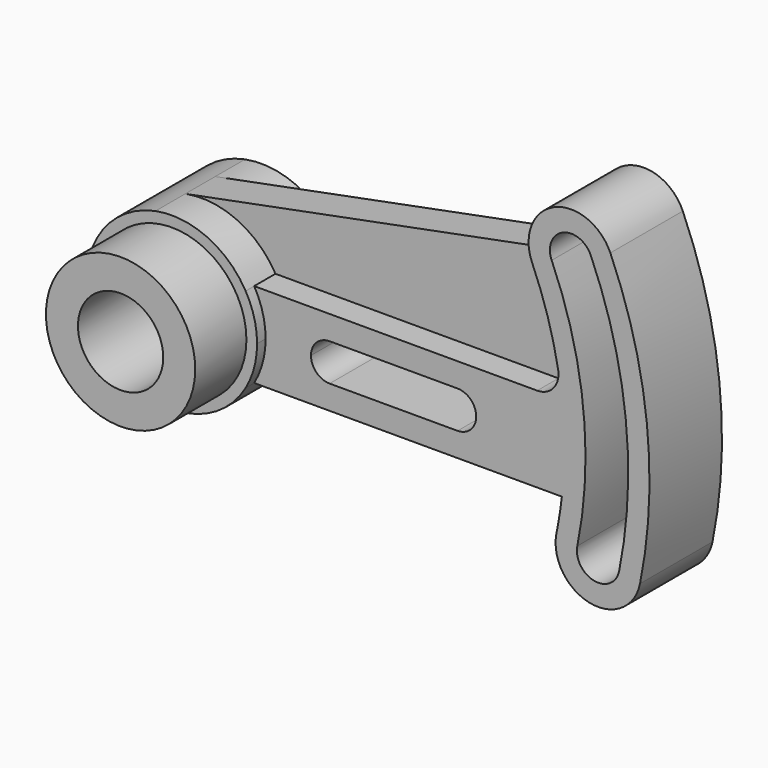
from build123d import *

# Parameters (mm, degrees)
F0_R     = 22.225
F1_DEPTH = 33.3248
F0_R_2   = 12.7
F2_DEPTH = 52.3748
F4_DEPTH = 3.175
F6_DEPTH = 3.175
F7_DEPTH = 22.225
F9_DEPTH = 11.0998


with BuildPart() as f1:
    # F0 (on Front) → F1 (new body)
    with BuildSketch(Plane.XZ):
        with BuildLine():
            ThreePointArc((21.9970452561, -12.7), (24.5345159877, -6.5740037456), (25.4, 0))
            ThreePointArc((25.4, 0), (24.5345159877, 6.5740037456), (21.9970452561, 12.7))
            ThreePointArc((21.9970452561, 12.7), (10.5332083635, 23.1130162803), (-4.8465484826, 24.9333304596))
            ThreePointArc((-4.8465484826, 24.9333304596), (-20.6785341663, -14.7498550751), (21.9970452561, -12.7))
        make_face()
        Circle(F0_R, mode=Mode.SUBTRACT)
        with BuildLine():
            ThreePointArc((21.9970452561, 12.7), (24.5345159877, 6.5740037456), (25.4, 0))
            ThreePointArc((25.4, 0), (24.5345159877, -6.5740037456), (21.9970452561, -12.7))
            Line((21.9970452561, -12.7), (44.45, -12.7))
            Line((44.45, -12.7), (113.592253257, -12.7))
            ThreePointArc((113.592253257, -12.7), (114.2376587708, 3.7745620369), (112.506165921, 20.1705882353))
            ThreePointArc((112.506165921, 20.1705882353), (111.126051049, 14.9752751807), (106.2558233698, 12.7))
            Line((106.2558233698, 12.7), (44.45, 12.7))
            Line((44.45, 12.7), (21.9970452561, 12.7))
        make_face()
        with BuildLine():
            ThreePointArc((44.45, -5.5499), (40.5256280751, -3.9243719249), (38.9001, 0))
            ThreePointArc((38.9001, 0), (40.5256280751, 3.9243719249), (44.45, 5.5499))
            Line((44.45, 5.5499), (82.55, 5.5499))
            ThreePointArc((82.55, 5.5499), (88.0999, 0), (82.55, -5.5499))
            Line((82.55, -5.5499), (44.45, -5.5499))
        make_face(mode=Mode.SUBTRACT)
        with BuildLine():
            ThreePointArc((112.506165921, 20.1705882353), (114.2376587708, 3.7745620369), (113.592253257, -12.7))
            ThreePointArc((113.592253257, -12.7), (112.9058029226, -17.7980242274), (111.99067104, -22.86))
            ThreePointArc((111.99067104, -22.86), (111.7983897902, -24.1235361825), (111.7340789334, -25.4))
            ThreePointArc((111.7340789334, -25.4), (123.1576151159, -38.0356891432), (136.8774868267, -27.94))
            ThreePointArc((136.8774868267, -27.94), (138.9294471202, 14.6526012321), (128.0371649171, 55.88))
            ThreePointArc((128.0371649171, 55.88), (113.9555393972, 63.2630335862), (103.7012522936, 51.1118625227))
            ThreePointArc((103.7012522936, 51.1118625227), (103.9343890657, 48.3581167453), (104.7576803867, 45.72))
            ThreePointArc((104.7576803867, 45.72), (109.380472839, 33.1723101625), (112.506165921, 20.1705882353))
        make_face()
        with BuildLine():
            ThreePointArc((130.6557828801, -26.67), (123.1640789334, -31.6217039467), (118.2123749867, -24.13))
            ThreePointArc((118.2123749867, -24.13), (119.9845225129, 12.6545192459), (110.5775515193, 48.26))
            ThreePointArc((110.5775515193, 48.26), (113.8574226519, 56.6198711326), (122.2172937845, 53.34))
            ThreePointArc((122.2172937845, 53.34), (132.6144722511, 13.9865739034), (130.6557828801, -26.67))
        make_face(mode=Mode.SUBTRACT)
    extrude(amount=F1_DEPTH)

    # F0 (on Front) → F2 (join)
    with BuildSketch(Plane.XZ):
        Circle(F0_R)
        Circle(F0_R_2, mode=Mode.SUBTRACT)
    extrude(amount=F2_DEPTH)

    # F3 (on face) → F4 (cut)
    with BuildSketch(Plane.XZ.offset(33.3248)):
        with BuildLine():
            ThreePointArc((21.9970452561, 12.7), (24.5345159877, 6.5740037456), (25.4, 0))
            ThreePointArc((25.4, 0), (24.5345159877, -6.5740037456), (21.9970452561, -12.7))
            Line((21.9970452561, -12.7), (113.592253257, -12.7))
            ThreePointArc((113.592253257, -12.7), (112.9058029226, -17.7980242274), (111.99067104, -22.86))
            ThreePointArc((111.99067104, -22.86), (121.8940789334, -37.8434078933), (136.8774868267, -27.94))
            ThreePointArc((136.8774868267, -27.94), (138.9294471202, 14.6526012321), (128.0371649171, 55.88))
            ThreePointArc((128.0371649171, 55.88), (111.3174226519, 62.4397422652), (104.7576803867, 45.72))
            ThreePointArc((104.7576803867, 45.72), (109.380472839, 33.1723101625), (112.506165921, 20.1705882353))
            ThreePointArc((112.506165921, 20.1705882353), (111.126051049, 14.9752751807), (106.2558233698, 12.7))
            Line((106.2558233698, 12.7), (21.9970452561, 12.7))
        make_face()
        with BuildLine():
            Line((82.55, -5.5499), (44.45, -5.5499))
            ThreePointArc((44.45, -5.5499), (38.9001, 0), (44.45, 5.5499))
            Line((44.45, 5.5499), (82.55, 5.5499))
            ThreePointArc((82.55, 5.5499), (88.0999, 0), (82.55, -5.5499))
        make_face(mode=Mode.SUBTRACT)
        with BuildLine():
            ThreePointArc((130.6557828801, -26.67), (123.1640789334, -31.6217039467), (118.2123749867, -24.13))
            ThreePointArc((118.2123749867, -24.13), (119.9845225129, 12.6545192459), (110.5775515193, 48.26))
            ThreePointArc((110.5775515193, 48.26), (113.8574226519, 56.6198711326), (122.2172937845, 53.34))
            ThreePointArc((122.2172937845, 53.34), (132.6144722511, 13.9865739034), (130.6557828801, -26.67))
        make_face(mode=Mode.SUBTRACT)
    extrude(amount=-F4_DEPTH, mode=Mode.SUBTRACT)

    # F5 (on face) → F6 (cut)
    with BuildSketch(Plane(origin=(0, 0, 0), x_dir=(-1, 0, 0), z_dir=(0, 1, 0))):
        with BuildLine():
            ThreePointArc((-21.9970452561, -12.7), (-25.4, 0), (-21.9970452561, 12.7))
            Line((-21.9970452561, 12.7), (-106.2558233698, 12.7))
            ThreePointArc((-106.2558233698, 12.7), (-111.126051049, 14.9752751807), (-112.506165921, 20.1705882353))
            ThreePointArc((-112.506165921, 20.1705882353), (-109.380472839, 33.1723101625), (-104.7576803867, 45.72))
            ThreePointArc((-104.7576803867, 45.72), (-111.3174226519, 62.4397422652), (-128.0371649171, 55.88))
            ThreePointArc((-128.0371649171, 55.88), (-138.9294471202, 14.6526012321), (-136.8774868267, -27.94))
            ThreePointArc((-136.8774868267, -27.94), (-121.8940789334, -37.8434078933), (-111.99067104, -22.86))
            ThreePointArc((-111.99067104, -22.86), (-112.9058029226, -17.7980242274), (-113.592253257, -12.7))
            Line((-113.592253257, -12.7), (-21.9970452561, -12.7))
        make_face()
        with BuildLine():
            ThreePointArc((-122.2172937845, 53.34), (-113.8574226519, 56.6198711326), (-110.5775515193, 48.26))
            ThreePointArc((-110.5775515193, 48.26), (-119.9845225129, 12.6545192459), (-118.2123749867, -24.13))
            ThreePointArc((-118.2123749867, -24.13), (-123.1640789334, -31.6217039467), (-130.6557828801, -26.67))
            ThreePointArc((-130.6557828801, -26.67), (-132.6144722511, 13.9865739034), (-122.2172937845, 53.34))
        make_face(mode=Mode.SUBTRACT)
        with BuildLine():
            Line((-82.55, 5.5499), (-44.45, 5.5499))
            ThreePointArc((-44.45, 5.5499), (-38.9001, 0), (-44.45, -5.5499))
            Line((-44.45, -5.5499), (-82.55, -5.5499))
            ThreePointArc((-82.55, -5.5499), (-88.0999, 0), (-82.55, 5.5499))
        make_face(mode=Mode.SUBTRACT)
    extrude(amount=-F6_DEPTH, mode=Mode.SUBTRACT)

    # F0 (on Front) → F7 (join)
    with BuildSketch(Plane.XZ):
        with BuildLine():
            ThreePointArc((-4.8465484826, 24.9333304596), (10.5332083635, 23.1130162803), (21.9970452561, 12.7))
            Line((21.9970452561, 12.7), (44.45, 12.7))
            Line((44.45, 12.7), (106.2558233698, 12.7))
            ThreePointArc((106.2558233698, 12.7), (111.126051049, 14.9752751807), (112.506165921, 20.1705882353))
            ThreePointArc((112.506165921, 20.1705882353), (109.380472839, 33.1723101625), (104.7576803867, 45.72))
            ThreePointArc((104.7576803867, 45.72), (103.9343890657, 48.3581167453), (103.7012522936, 51.1118625227))
            ThreePointArc((103.7012522936, 51.1118625227), (102.2030178457, 47.1688368577), (98.5648042351, 45.0344611692))
            Line((98.5648042351, 45.0344611692), (-4.8465484826, 24.9333304596))
        make_face()
    extrude(amount=F7_DEPTH)

    # F8 (on face) → F9 (cut)
    with BuildSketch(Plane(origin=(0, 0, 0), x_dir=(-1, 0, 0), z_dir=(0, 1, 0))):
        with BuildLine():
            ThreePointArc((-21.9970452561, 12.7), (-10.5332083635, 23.1130162803), (4.8465484826, 24.9333304596))
            Line((4.8465484826, 24.9333304596), (-98.5648042351, 45.0344611692))
            ThreePointArc((-98.5648042351, 45.0344611692), (-102.2030178457, 47.1688368577), (-103.7012522936, 51.1118625227))
            ThreePointArc((-103.7012522936, 51.1118625227), (-103.9343890657, 48.3581167453), (-104.7576803867, 45.72))
            ThreePointArc((-104.7576803867, 45.72), (-109.380472839, 33.1723101625), (-112.506165921, 20.1705882353))
            ThreePointArc((-112.506165921, 20.1705882353), (-111.126051049, 14.9752751807), (-106.2558233698, 12.7))
            Line((-106.2558233698, 12.7), (-21.9970452561, 12.7))
        make_face()
    extrude(amount=-F9_DEPTH, mode=Mode.SUBTRACT)


solid = f1.part
